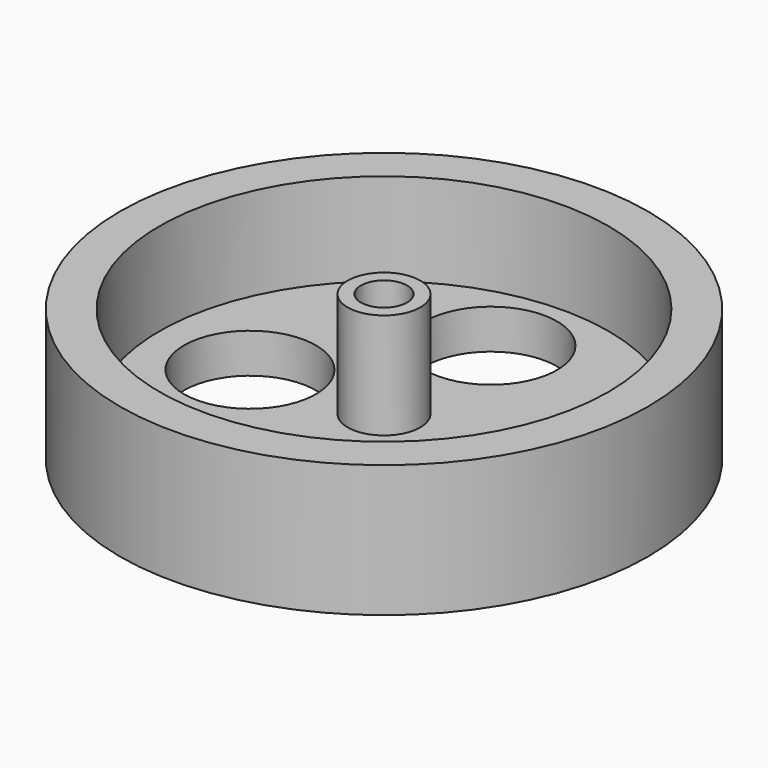
from build123d import *

# Parameters (mm, degrees)
F0_R     = 20
F1_DEPTH = 10
F2_T     = -3
F6_R     = 2.75
F7_DEPTH = 8
F9_D     = 3.5
F11_D    = 10
F13_D    = 10
F15_D    = 10
F17_D    = 10


# Not quite as in the source:
# - the program builds the solid bodies; features that only make, move or delete a surface that nothing else refers to are left out


with BuildPart() as f1:
    # F0 (on Top) → F1 (new body)
    with BuildSketch(Plane.XY):
        Circle(F0_R)
    extrude(amount=-F1_DEPTH)

    # F2
    f2_openings = [f1.faces().sort_by_distance(p)[0] for p in [
        (0, 0, 0),
    ]]
    offset(amount=F2_T, openings=f2_openings)

    # F6 (on face) → F7 (join)
    with BuildSketch(Plane.XY.offset(-7)):
        Circle(F6_R)
    extrude(amount=F7_DEPTH)

    # F9 (through all)
    with Locations(Plane.XY.offset(1)):
        with Locations((0, 0)):
            Hole(F9_D / 2)

    # F11 (through all)
    with Locations(Plane.XY):
        with Locations((-0.525876123, 10.7804676518)):
            Hole(F11_D / 2)

    # F13 (through all)
    with Locations(Plane.XY):
        with Locations((-9.7287148237, -0.5258764722)):
            Hole(F13_D / 2)

    # F15 (through all)
    with Locations(Plane.XY):
        with Locations((0.5258767051, -11.0434060916)):
            Hole(F15_D / 2)

    # F17 (through all)
    with Locations(Plane.XY):
        with Locations((11.3063445315, -0.7888147375)):
            Hole(F17_D / 2)


solid = f1.part
